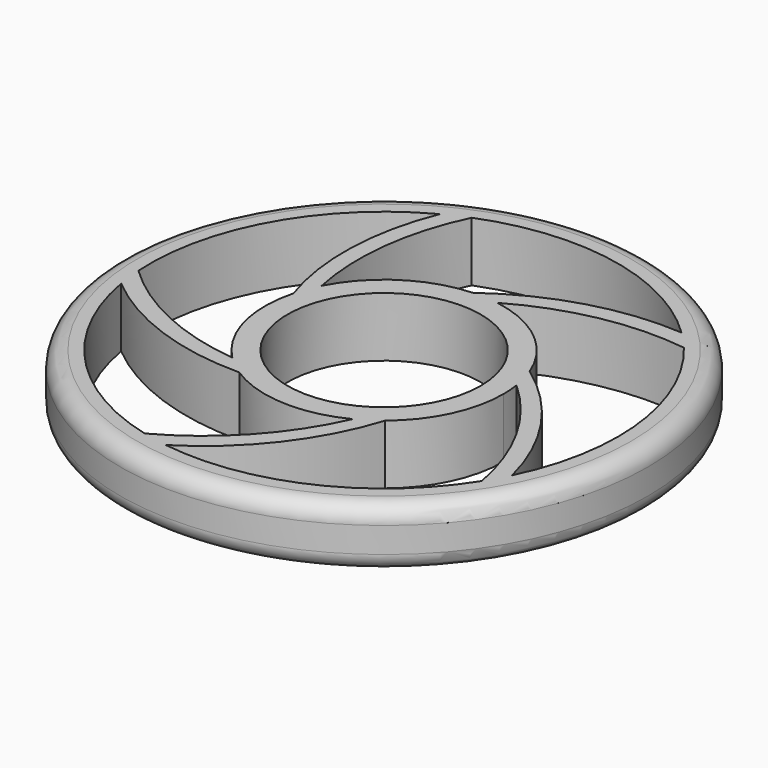
from build123d import *

# Parameters (mm, degrees)
F0_R     = 31
F0_R_2   = 11.35
F1_DEPTH = 7
F2_R     = 2


# Not quite as in the source:
# - a feature names something its author has since deleted; it is built from what else it names


with BuildPart() as f1:
    # F0 (on Top) → F1 (new body)
    with BuildSketch(Plane.XY):
        Circle(F0_R)
        with BuildLine():
            ThreePointArc((21.1666938057, 17.5562260562), (25.8682631776, 9.3318251254), (27.5, 0))
            ThreePointArc((27.5, 0), (26.7912185144, -6.2032741767), (24.7014101446, -12.0867835617))
            ThreePointArc((24.7014101446, -12.0867835617), (24.0053577694, -13.4161394731), (23.237831293, -14.7055498639))
            ThreePointArc((23.237831293, -14.7055498639), (11.5349334666, -24.9638801055), (-3.8620587477, -27.2274586076))
            ThreePointArc((-3.8620587477, -27.2274586076), (-5.3414433626, -26.9762670287), (-6.8049242418, -26.6447556953))
            ThreePointArc((-6.8049242418, -26.6447556953), (-20.1775703762, -18.6846368365), (-27.0882937172, -4.740711285))
            ThreePointArc((-27.0882937172, -4.740711285), (-27.3065513165, -3.2561104403), (-27.4435057653, -1.7618147778))
            ThreePointArc((-27.4435057653, -1.7618147778), (-24.0053577694, 13.4161394731), (-12.8794274668, 24.2975379026))
            ThreePointArc((-12.8794274668, 24.2975379026), (-11.5349334666, 24.9638801055), (-10.1560950916, 25.5558942808))
            ThreePointArc((-10.1560950916, 25.5558942808), (5.3414433626, 26.9762670287), (19.1283697872, 19.7574155518))
            ThreePointArc((19.1283697872, 19.7574155518), (20.1775703762, 18.6846368365), (21.1666938057, 17.5562260562))
        make_face(mode=Mode.SUBTRACT)
        with BuildLine():
            ThreePointArc((13.0616927236, 5.0390657066), (8.8208386376, 10.871651472), (2.2395865353, 13.8197052122))
            ThreePointArc((2.2395865353, 13.8197052122), (0.7460119592, 13.9801096618), (-0.7561512494, 13.9795649177))
            ThreePointArc((-0.7561512494, 13.9795649177), (-7.6137659317, 11.7486411273), (-12.4512503955, 6.400497136))
            ThreePointArc((-12.4512503955, 6.400497136), (-13.065344019, 5.0295910037), (-13.5290198963, 3.6007805605))
            ThreePointArc((-13.5290198963, 3.6007805605), (-13.5264047658, -3.6105919337), (-9.9348824822, -9.8639804372))
            ThreePointArc((-9.9348824822, -9.8639804372), (-8.8208386376, -10.871651472), (-7.605242881, -11.7541601453))
            ThreePointArc((-7.605242881, -11.7541601453), (-0.7460119592, -13.9801096618), (6.3111553473, -12.4967723106))
            ThreePointArc((6.3111553473, -12.4967723106), (7.6137659317, -11.7486411273), (8.8287213032, -10.8652510395))
            ThreePointArc((8.8287213032, -10.8652510395), (12.6412439705, -6.016556397), (14, 0))
            ThreePointArc((14, 0), (13.9587870879, 1.0734351561), (13.8353909951, 2.1405503996))
            ThreePointArc((13.8353909951, 2.1405503996), (13.5264047658, 3.6105919337), (13.0616927236, 5.0390657066))
        make_face()
        Circle(F0_R_2, mode=Mode.SUBTRACT)
        with BuildLine():
            ThreePointArc((2.2395865353, 13.8197052122), (11.3945871221, 17.2509213593), (21.1666938057, 17.5562260562))
            ThreePointArc((21.1666938057, 17.5562260562), (20.1775703762, 18.6846368365), (19.1283697872, 19.7574155518))
            ThreePointArc((19.1283697872, 19.7574155518), (8.6718028957, 18.6384798978), (-0.7561512494, 13.9795649177))
            ThreePointArc((-0.7561512494, 13.9795649177), (0.7460119592, 13.9801096618), (2.2395865353, 13.8197052122))
        make_face()
        with BuildLine():
            ThreePointArc((-12.4512503955, 6.400497136), (-12.8854801062, 16.1677242016), (-10.1560950916, 25.5558942808))
            ThreePointArc((-10.1560950916, 25.5558942808), (-11.5349334666, 24.9638801055), (-12.8794274668, 24.2975379026))
            ThreePointArc((-12.8794274668, 24.2975379026), (-15.046513294, 14.0069816897), (-13.5290198963, 3.6007805605))
            ThreePointArc((-13.5290198963, 3.6007805605), (-13.065344019, 5.0295910037), (-12.4512503955, 6.400497136))
        make_face()
        with BuildLine():
            ThreePointArc((-9.9348824822, -9.8639804372), (-19.3582517891, -7.258718282), (-27.4435057653, -1.7618147778))
            ThreePointArc((-27.4435057653, -1.7618147778), (-27.3065513165, -3.2561104403), (-27.0882937172, -4.740711285))
            ThreePointArc((-27.0882937172, -4.740711285), (-17.9710595236, -9.9816891338), (-7.605242881, -11.7541601453))
            ThreePointArc((-7.605242881, -11.7541601453), (-8.8208386376, -10.871651472), (-9.9348824822, -9.8639804372))
        make_face()
        with BuildLine():
            ThreePointArc((-6.8049242418, -26.6447556953), (-5.3414433626, -26.9762670287), (-3.8620587477, -27.2274586076))
            ThreePointArc((-3.8620587477, -27.2274586076), (3.9397876946, -20.1760048395), (8.8287213032, -10.8652510395))
            ThreePointArc((8.8287213032, -10.8652510395), (7.6137659317, -11.7486411273), (6.3111553473, -12.4967723106))
            ThreePointArc((6.3111553473, -12.4967723106), (0.9214225378, -20.6538588146), (-6.8049242418, -26.6447556953))
        make_face()
        with BuildLine():
            ThreePointArc((23.237831293, -14.7055498639), (24.0053577694, -13.4161394731), (24.7014101446, -12.0867835617))
            ThreePointArc((24.7014101446, -12.0867835617), (20.4059822273, -2.4877676142), (13.0616927236, 5.0390657066))
            ThreePointArc((13.0616927236, 5.0390657066), (13.5264047658, 3.6105919337), (13.8353909951, 2.1405503996))
            ThreePointArc((13.8353909951, 2.1405503996), (19.9277222355, -5.5060684643), (23.237831293, -14.7055498639))
        make_face()
    extrude(amount=F1_DEPTH)

    # F2
    f2_edges = [f1.edges().sort_by_distance(p)[0] for p in [
        (-31, 0, 7),
        (-31, 0, 0),
    ]]
    fillet(f2_edges, radius=F2_R)


solid = f1.part
